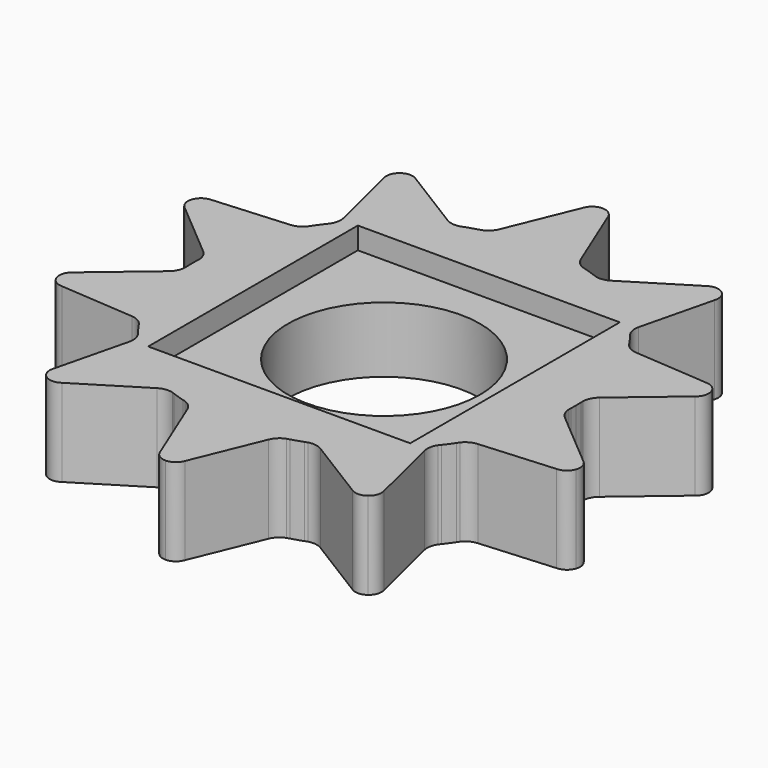
from build123d import *

# Parameters (mm, degrees)
F1_DEPTH        = 1
F1_COPIES_COUNT = 10
F3_W            = 3
F3_H            = 3
F4_DEPTH        = 0.25
F5_DEPTH        = 1
F6_DEPTH        = 0.25
F7_R            = 1.1
F8_DEPTH        = 1.31


# Not quite as in the source:
# - ends of sketch curves that miss each other by under 0.0002 mm in the source are joined
# - a feature of the source that left no trace in its solid (it failed there, or was rolled back) is left out
# - a pattern or mirror of a feature is missing from the dataset's text; its kind, count and spacing are read off the source's solid


with BuildPart() as f1:
    # F0 (on Top) → F1 (new body)
    with BuildSketch(Plane.XY):
        with BuildLine():
            ThreePointArc((0.581444512, 2.1217733808), (0.2933415776, 2.1803556405), (0, 2.2))
            ThreePointArc((0, 2.2), (-0.2933416878, 2.1803556256), (-0.5814447265, 2.121773322))
            ThreePointArc((-0.5814447265, 2.121773322), (-0.5968372157, 2.1167523736), (-0.6125853979, 2.1129929319))
            ThreePointArc((-0.6125853979, 2.1129929319), (-1.3214219849, -1.7589326132), (2.2, 0))
            ThreePointArc((2.2, 0), (1.7589325969, 1.3214220066), (0.612585346, 2.112992947))
            ThreePointArc((0.6125853416, 2.1129929319), (0.5968370782, 2.1167523965), (0.581444512, 2.1217733808))
        make_face()
        with BuildLine():
            ThreePointArc((0.6, 0.8), (0, -1), (-0.6, 0.8))
            Line((-0.6, 0.8), (0, 0.8))
            Line((0, 0.8), (0.6, 0.8))
        make_face(mode=Mode.SUBTRACT)
        with BuildLine():
            ThreePointArc((-0.5814447265, 2.121773322), (-0.2933416878, 2.1803556256), (0, 2.2))
            Line((0, 2.2), (0, 2.8273255734))
            ThreePointArc((0, 2.8273255734), (-0.1215931939, 2.889819495), (-0.1419835484, 3.0250031792))
            Line((-0.1419835484, 3.0250031792), (-0.4660251262, 2.233467269))
            ThreePointArc((-0.4660251262, 2.233467269), (-0.5120300634, 2.1655250062), (-0.5814447265, 2.121773322))
        make_face()
        with BuildLine():
            Line((0, 2.8273255734), (0, 2.2))
            ThreePointArc((0, 2.2), (0.2933415776, 2.1803556405), (0.581444512, 2.1217733808))
            ThreePointArc((0.581444512, 2.1217733808), (0.5119904355, 2.165563311), (0.4659834267, 2.2335690598))
            Line((0.4659834267, 2.2335690598), (0.1424618925, 3.0249932315))
            ThreePointArc((0.1424618925, 3.0249932315), (0.1482808399, 3.0014743175), (0.1502375048, 2.9773253853))
            ThreePointArc((0.1502375048, 2.9773253853), (0.1062195181, 2.8711754307), (0, 2.8273255734))
        make_face()
        with BuildLine():
            ThreePointArc((-0.1419835484, 3.0250031792), (-0.1215931939, 2.889819495), (0, 2.8273255734))
            Line((0, 2.8273255734), (0, 3.1273251973))
            ThreePointArc((0, 3.1273251973), (-0.0874611784, 3.0990173775), (-0.1419835484, 3.0250031792))
        make_face()
        with BuildLine():
            Line((0, 3.1273251973), (0, 2.8273255734))
            ThreePointArc((0, 2.8273255734), (0.1062195181, 2.8711754307), (0.1502375048, 2.9773253853))
            ThreePointArc((0.1502375048, 2.9773253853), (0.1482808399, 3.0014743175), (0.1424618925, 3.0249932315))
            ThreePointArc((0.1424618925, 3.0249932315), (0.0877476558, 3.0991530237), (0, 3.1273251973))
        make_face()
        with BuildLine():
            ThreePointArc((0.612585346, 2.112992947), (0.5970310708, 2.1174404125), (0.581444512, 2.1217733808))
            ThreePointArc((0.581444512, 2.1217733808), (0.5968370782, 2.1167523965), (0.6125853416, 2.1129929319))
        make_face()
        with BuildLine():
            ThreePointArc((-0.6125853979, 2.1129929319), (-0.5968372157, 2.1167523736), (-0.5814447265, 2.121773322))
            ThreePointArc((-0.5814447265, 2.121773322), (-0.5970312038, 2.117440375), (-0.6125853979, 2.1129929319))
        make_face()
    extrude(amount=F1_DEPTH)

    # F1_copies: F1 ×10 about axis
    f1_copies_axis = Axis((0, 0, 0), (0, 0, 1))


with BuildPart() as f1_1:
    add(f1.part)
    for i in range(1, F1_COPIES_COUNT):
        add(f1.part.rotate(f1_copies_axis, i * 360 / F1_COPIES_COUNT))

    # F3 (on face) → F4 (cut)
    with BuildSketch(Plane.XY.offset(1)):
        Rectangle(F3_W, F3_H)
    extrude(amount=-F4_DEPTH, mode=Mode.SUBTRACT)

    # F0 (on Top) → F5 (join)
    with BuildSketch(Plane.XY):
        with BuildLine():
            ThreePointArc((0.581444512, 2.1217733808), (0.2933415776, 2.1803556405), (0, 2.2))
            ThreePointArc((0, 2.2), (-0.2933416878, 2.1803556256), (-0.5814447265, 2.121773322))
            ThreePointArc((-0.5814447265, 2.121773322), (-0.5968372157, 2.1167523736), (-0.6125853979, 2.1129929319))
            ThreePointArc((-0.6125853979, 2.1129929319), (-1.3214219849, -1.7589326132), (2.2, 0))
            ThreePointArc((2.2, 0), (1.7589325969, 1.3214220066), (0.612585346, 2.112992947))
            ThreePointArc((0.6125853416, 2.1129929319), (0.5968370782, 2.1167523965), (0.581444512, 2.1217733808))
        make_face()
        with BuildLine():
            ThreePointArc((0.6, 0.8), (0, -1), (-0.6, 0.8))
            Line((-0.6, 0.8), (0, 0.8))
            Line((0, 0.8), (0.6, 0.8))
        make_face(mode=Mode.SUBTRACT)
        with BuildLine():
            ThreePointArc((-0.5814447265, 2.121773322), (-0.2933416878, 2.1803556256), (0, 2.2))
            Line((0, 2.2), (0, 2.8273255734))
            ThreePointArc((0, 2.8273255734), (-0.1215931939, 2.889819495), (-0.1419835484, 3.0250031792))
            Line((-0.1419835484, 3.0250031792), (-0.4660251262, 2.233467269))
            ThreePointArc((-0.4660251262, 2.233467269), (-0.5120300634, 2.1655250062), (-0.5814447265, 2.121773322))
        make_face()
        with BuildLine():
            Line((0, 2.8273255734), (0, 2.2))
            ThreePointArc((0, 2.2), (0.2933415776, 2.1803556405), (0.581444512, 2.1217733808))
            ThreePointArc((0.581444512, 2.1217733808), (0.5119904355, 2.165563311), (0.4659834267, 2.2335690598))
            Line((0.4659834267, 2.2335690598), (0.1424618925, 3.0249932315))
            ThreePointArc((0.1424618925, 3.0249932315), (0.1482808399, 3.0014743175), (0.1502375048, 2.9773253853))
            ThreePointArc((0.1502375048, 2.9773253853), (0.1062195181, 2.8711754307), (0, 2.8273255734))
        make_face()
        with BuildLine():
            ThreePointArc((-0.1419835484, 3.0250031792), (-0.1215931939, 2.889819495), (0, 2.8273255734))
            Line((0, 2.8273255734), (0, 3.1273251973))
            ThreePointArc((0, 3.1273251973), (-0.0874611784, 3.0990173775), (-0.1419835484, 3.0250031792))
        make_face()
        with BuildLine():
            Line((0, 3.1273251973), (0, 2.8273255734))
            ThreePointArc((0, 2.8273255734), (0.1062195181, 2.8711754307), (0.1502375048, 2.9773253853))
            ThreePointArc((0.1502375048, 2.9773253853), (0.1482808399, 3.0014743175), (0.1424618925, 3.0249932315))
            ThreePointArc((0.1424618925, 3.0249932315), (0.0877476558, 3.0991530237), (0, 3.1273251973))
        make_face()
        with BuildLine():
            ThreePointArc((0.612585346, 2.112992947), (0.5970310708, 2.1174404125), (0.581444512, 2.1217733808))
            ThreePointArc((0.581444512, 2.1217733808), (0.5968370782, 2.1167523965), (0.6125853416, 2.1129929319))
        make_face()
        with BuildLine():
            ThreePointArc((-0.6125853979, 2.1129929319), (-0.5968372157, 2.1167523736), (-0.5814447265, 2.121773322))
            ThreePointArc((-0.5814447265, 2.121773322), (-0.5970312038, 2.117440375), (-0.6125853979, 2.1129929319))
        make_face()
    extrude(amount=F5_DEPTH)

    # F3 (on face) → F6 (cut)
    with BuildSketch(Plane.XY.offset(1)):
        Rectangle(F3_W, F3_H)
        Polygon((-0.259935757, 0.8), (0.259935757, 0.8), (0.6805206467, 0.494427191), (0.8411697794, 0), (0.6805206467, -0.494427191), (0.259935757, -0.8), (-0.259935757, -0.8), (-0.6805206467, -0.494427191), (-0.8411697794, 0), (-0.6805206467, 0.494427191), align=None, mode=Mode.SUBTRACT)
    extrude(amount=-F6_DEPTH, mode=Mode.SUBTRACT)

    # F7 (on face) → F8 (cut, symmetric)
    with BuildSketch(Plane.XY.offset(1)):
        Circle(F7_R)
    extrude(amount=F8_DEPTH, both=True, mode=Mode.SUBTRACT)


solid = f1_1.part
